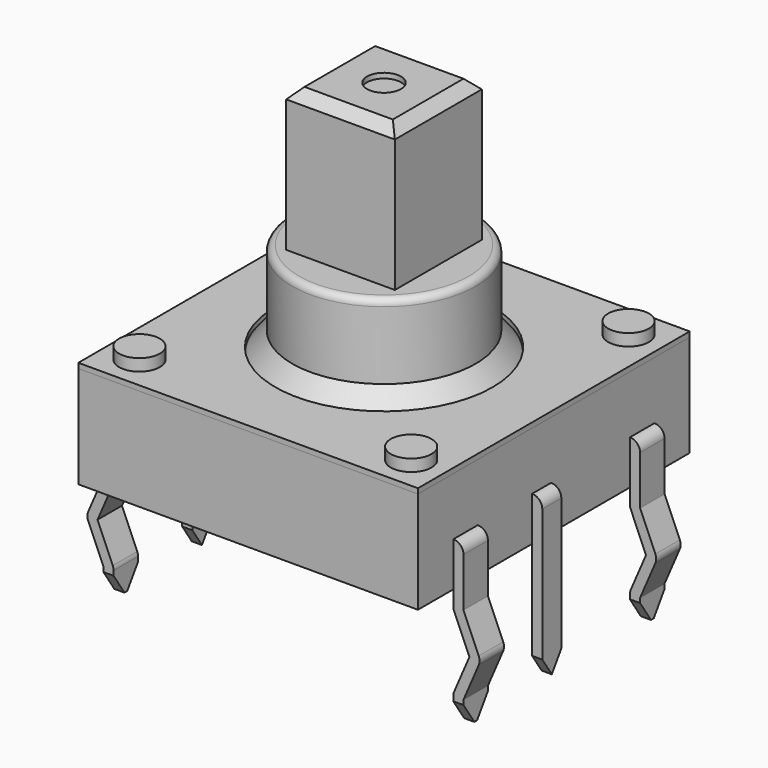
from build123d import *

# Parameters (mm, degrees)
F0_W           = 10
F0_H           = 10
F1_DEPTH       = 3
F2_W           = 10
F2_H           = 10
F2_R           = 0.6
F2_R_2         = 3.2
F3_DEPTH       = 0.15
F4_DEPTH       = 0.5
F5_W           = 2.7
F5_H           = 2.2041232037
F7_W           = 3.2
F7_H           = 3.2
F8_DEPTH       = 4.2
F9_R           = 0.5
F10_DEPTH      = 0.15
F11_SIZE       = 0.3
F12_R          = 0.2
F15_DEPTH      = 0.45
F17_W          = 0.3
F17_H          = 4.8
F18_DEPTH      = 0.35
F19_C1_SIZE2   = 0.6
F19_C1_SIZE    = 0.4
F19_C2_SIZE2   = 0.6
F19_C2_SIZE    = 0.4
F19_2_T1_DEPTH = 3.4005606286
F20_R          = 0.29999
F20_2_R        = 0.29999


# Not quite as in the source:
# - a fillet or chamfer that OpenCascade refuses, or shapes differently, is made with other operations: its cross-section is extruded or revolved along the edge and cut away or added
# - a fillet or chamfer is up to 0.001 mm smaller than in the source, because OpenCascade refuses the exact size


with BuildPart() as f1:
    # F0 (on Top) → F1 (new body)
    with BuildSketch(Plane.XY):
        Rectangle(F0_W, F0_H)
    extrude(amount=F1_DEPTH)

    # F2 (on face) → F4 (join)
    with BuildSketch(Plane.XY.offset(3)):
        with Locations((-4, 4)):
            Circle(F2_R)
        with Locations((4, -4)):
            Circle(F2_R)
        with Locations((4, 4)):
            Circle(F2_R)
        with Locations((-4, -4)):
            Circle(F2_R)
    extrude(amount=F4_DEPTH)

    # F5 (on Front) → F6 (revolve)
    with BuildSketch(Plane.XZ):
        Polygon((-3.2, 3), (0, 3), (0, 3.5958767963), (-2.7, 3.5958767963), align=None)
        with Locations((-1.35, 4.6979383981)):
            Rectangle(F5_W, F5_H)
    revolve(axis=Axis((0, 0, 4.6979383981), (0, 0, -1)))

    # F7 (on face) → F8 (join)
    with BuildSketch(Plane.XY.offset(5.8)):
        Rectangle(F7_W, F7_H)
    extrude(amount=F8_DEPTH)

    # F9 (on face) → F10 (cut)
    with BuildSketch(Plane.XY.offset(10)):
        Circle(F9_R)
    extrude(amount=-F10_DEPTH, mode=Mode.SUBTRACT)

    # F11
    f11_edges = [f1.edges().sort_by_distance(p)[0] for p in [
        (-1.6, 0, 10),
        (0, -1.6, 10),
        (1.6, 0, 10),
        (0, 1.6, 10),
    ]]
    chamfer(f11_edges, length=F11_SIZE)

    # F12
    f12_edges = [f1.edges().sort_by_distance(p)[0] for p in [
        (2.7, 0, 5.8),
    ]]
    fillet(f12_edges, radius=F12_R)


with BuildPart() as f3:
    # F2 (on face) → F3 (new body)
    with BuildSketch(Plane.XY.offset(3)):
        Rectangle(F2_W, F2_H)
        with Locations((-4, -4)):
            Circle(F2_R, mode=Mode.SUBTRACT)
        with Locations((4, -4)):
            Circle(F2_R, mode=Mode.SUBTRACT)
        with Locations((-4, 4)):
            Circle(F2_R, mode=Mode.SUBTRACT)
        Circle(F2_R_2, mode=Mode.SUBTRACT)
        with Locations((4, 4)):
            Circle(F2_R, mode=Mode.SUBTRACT)
    extrude(amount=F3_DEPTH)


with BuildPart() as f15:
    # F14 (on offset) → F15 (new body, symmetric)
    with BuildSketch(Plane.XZ.offset(3.25)):
        Polygon((-5, -0.5), (-5, 1.3), (-5.3, 1.3), (-5.3, -0.4381863865), (-5.8, -1.6), (-5.3, -2.7618136135), (-5.3, -3.5), (-5, -3.5), (-5, -2.7), (-5.4733977926, -1.6), align=None)
    extrude(amount=F15_DEPTH, both=True)

    # F19: chamfer of 0.4 x 0.6 on 2 edges, made by hand

    # F19_c1
    f19_c1_edges = [f15.edges().sort_by_distance(p)[0] for p in [
        (-5.15, -2.8, -3.5),
    ]]
    f19_c1_side = f15.faces().sort_by_distance((-5.15, -2.808, -3.5))[0]
    chamfer(f19_c1_edges, length=F19_C1_SIZE, length2=F19_C1_SIZE2, reference=f19_c1_side)

    # F19_c2
    f19_c2_edges = [f15.edges().sort_by_distance(p)[0] for p in [
        (-5.15, -3.7, -3.5),
    ]]
    f19_c2_side = f15.faces().sort_by_distance((-5.15, -3.692, -3.5))[0]
    chamfer(f19_c2_edges, length=F19_C2_SIZE, length2=F19_C2_SIZE2, reference=f19_c2_side)

    # F20 (radius 0.3 in the source; OpenCascade refuses exactly that, so slightly less here)
    f20_edges = [f15.edges().sort_by_distance(p)[0] for p in [
        (-5.8, -3.25, -1.6),
        (-5.3, -3.25, 1.3),
        (-5, -3.25, -2.7),
        (-5, -3.25, -0.5),
    ]]
    fillet(f20_edges, radius=F20_R)


with BuildPart() as f18:
    # F17 (on offset) → F18 (new body, symmetric)
    with BuildSketch(Plane.XZ.offset(0.45)):
        with Locations((-5.15, -1.1)):
            Rectangle(F17_W, F17_H)
    extrude(amount=F18_DEPTH, both=True)

    # F19#2: chamfer of 0.4 x 0.6 on 2 edges, made by hand

    # F19_2_s2 → F19_2_t1 (cut)
    with BuildSketch(Plane.YZ.offset(-6.8502803143)):
        Polygon((-0.4, -3.5), (-0.8, -2.9), (-0.8, -3.5), align=None)
        Polygon((-0.5, -3.5), (-0.1, -2.9), (-0.1, -3.5), align=None)
    extrude(amount=F19_2_T1_DEPTH, mode=Mode.SUBTRACT)

    # F20#2 (radius 0.3 in the source; OpenCascade refuses exactly that, so slightly less here)
    f20_2_edges = [f18.edges().sort_by_distance(p)[0] for p in [
        (-5.3, -0.45, 1.3),
    ]]
    fillet(f20_2_edges, radius=F20_2_R)


with BuildPart() as f21_1:
    # F21: instance of F15
    add(f15.part.mirror(Plane.XZ))


with BuildPart() as f22_1:
    # F22: instance of F21_1
    add(f21_1.part.mirror(Plane.YZ))


with BuildPart() as f22_2:
    # F22: instance of F15
    add(f15.part.mirror(Plane.YZ))


with BuildPart() as f22_3:
    # F22: instance of F18
    add(f18.part.mirror(Plane.YZ))


solid = Compound([f1.part, f3.part, f15.part, f18.part, f21_1.part, f22_1.part, f22_2.part, f22_3.part])
